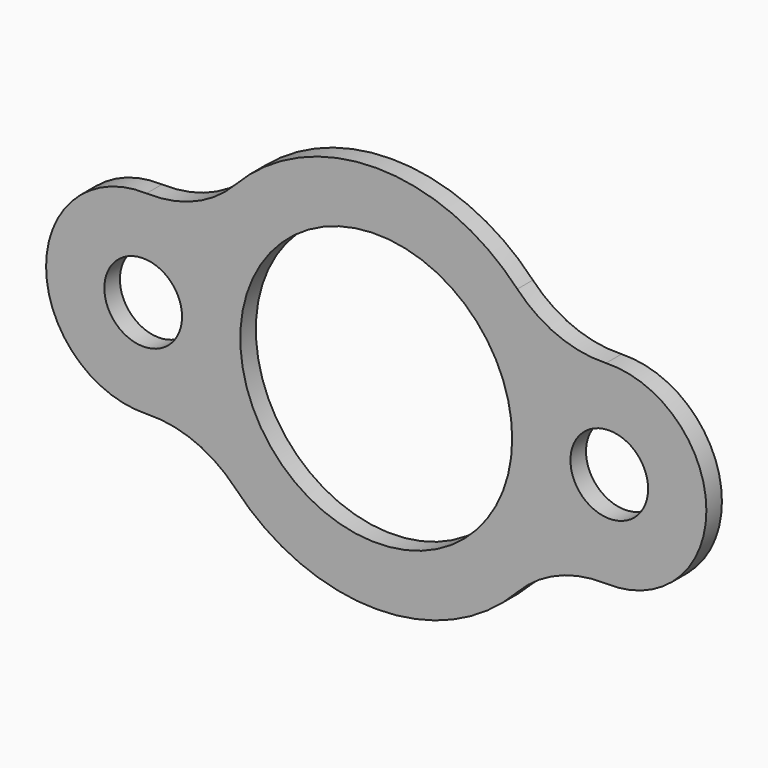
from build123d import *

# Parameters (mm, degrees)
F0_R     = 12.7
F0_R_2   = 44.45
F1_DEPTH = 6.35


# Not quite as in the source:
# - a length typed as a fraction of an inch, garbled in the dataset ("3 / 203.2 mm" for 3/8 in), is restored


with BuildPart() as f1:
    # F0 (on Front) → F1 (new body)
    with BuildSketch(Plane.XZ):
        with BuildLine():
            ThreePointArc((-46.13671875, 43.6308741946), (-59.3475236203, 34.5646316236), (-75.1176136364, 31.7315448688))
            ThreePointArc((-75.1176136364, 31.7315448688), (-107.95, 0), (-75.1176136364, -31.7315448688))
            ThreePointArc((-75.1176136364, -31.7315448688), (-59.3475236203, -34.5646316236), (-46.13671875, -43.6308741946))
            ThreePointArc((-46.13671875, -43.6308741946), (0, -63.5), (46.13671875, -43.6308741946))
            ThreePointArc((46.13671875, -43.6308741946), (59.3475236203, -34.5646316236), (75.1176136364, -31.7315448688))
            ThreePointArc((75.1176136364, -31.7315448688), (107.95, 0), (75.1176136364, 31.7315448688))
            ThreePointArc((75.1176136364, 31.7315448688), (59.3475236203, 34.5646316236), (46.13671875, 43.6308741946))
            ThreePointArc((46.13671875, 43.6308741946), (0, 63.5), (-46.13671875, 43.6308741946))
        make_face()
        with Locations((-76.2, 0)):
            Circle(F0_R, mode=Mode.SUBTRACT)
        Circle(F0_R_2, mode=Mode.SUBTRACT)
        with Locations((76.2, 0)):
            Circle(F0_R, mode=Mode.SUBTRACT)
    extrude(amount=F1_DEPTH)


solid = f1.part
